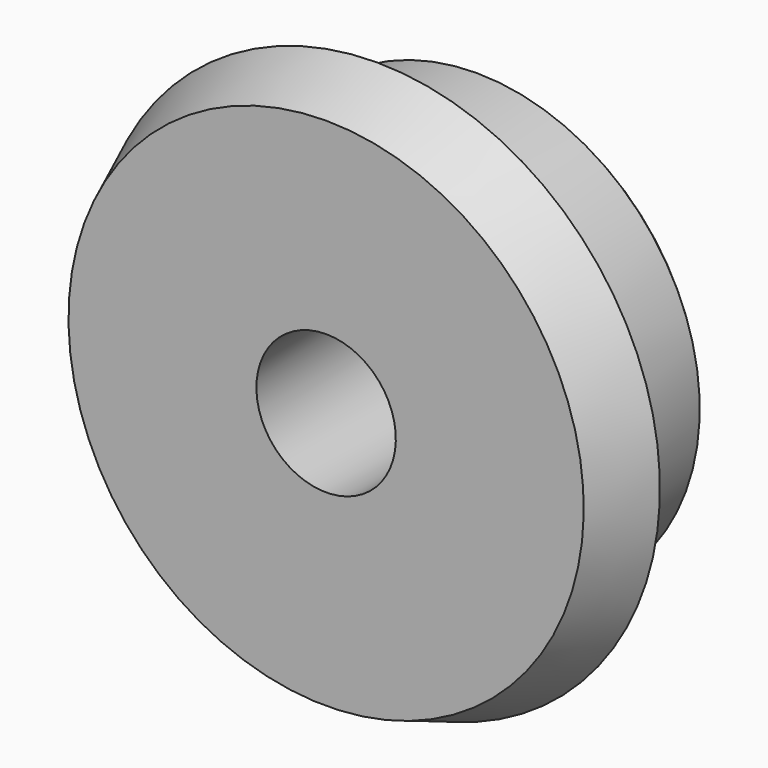
from build123d import *

# Parameters (mm, degrees)
F0_W    = 15.0114
F0_H    = 17.4625
F0_W_2  = 7.2136
F0_H_2  = 10.287
F2_R    = 1.5875
F3_SIZE = 0.79375


# Not quite as in the source:
# - a fillet or chamfer that OpenCascade refuses, or shapes differently, is made with other operations: its cross-section is extruded or revolved along the edge and cut away or added


with BuildPart() as f1:
    # F0 (on Right) → F1 (revolve)
    with BuildSketch(Plane.YZ):
        with Locations((14.7193, 16.66875)):
            Rectangle(F0_W, F0_H)
        with Locations((3.6068, 16.66875)):
            Rectangle(F0_W_2, F0_H)
        with Locations((3.6068, 30.5435)):
            Rectangle(F0_W_2, F0_H_2)
    revolve(axis=Axis((0, 11.1125, 0), (0, 1, 0)))

    # F2
    f2_edges = [f1.edges().sort_by_distance(p)[0] for p in [
        (0, 7.2136, -25.4),
    ]]
    fillet(f2_edges, radius=F2_R)

    # F3
    f3_edges = [f1.edges().sort_by_distance(p)[0] for p in [
        (0, 22.225, -25.4),
    ]]
    chamfer(f3_edges, length=F3_SIZE)

    # F4: chamfer of 6.35 x 15.748 on 2 edges, made by hand

    # F4_s1 → F4_t2 (revolve, cut)
    with BuildSketch(Plane.YZ):
        Polygon((15.748, 35.687), (0, 29.337), (0, 35.687), align=None)
    revolve(axis=Axis((0, 0, 0), (0, 1, 0)), mode=Mode.SUBTRACT)


solid = f1.part
